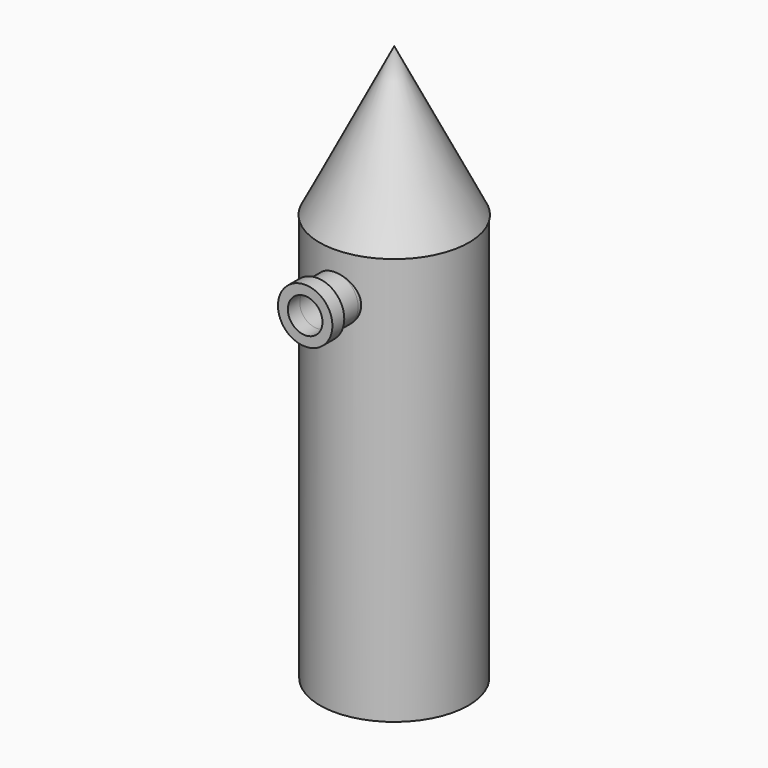
from build123d import *

# Parameters (mm, degrees)
F1_R      = 6.35
F2_DEPTH  = 0.127
F0_R      = 25.4
F3_DEPTH  = 69.85
F6_R      = 6.4657845793
F7_DEPTH  = 152.4
F9_R      = 5.9402933738
F10_DEPTH = 12.7
F9_R_2    = 7.9512438963
F11_DEPTH = 12.7
F12_R     = 9.3192729134
F12_R_2   = 5.9212982026
F13_DEPTH = 5.08
F14_DEPTH = 2.54


with BuildPart() as f2:
    # F1 (on Top) → F2 (new body, symmetric)
    with BuildSketch(Plane.XY):
        Circle(F1_R)
    extrude(amount=F2_DEPTH, both=True)


with BuildPart() as f3:
    # F0 (on Top) → F3 (new body, symmetric)
    with BuildSketch(Plane.XY):
        Circle(F0_R)
    extrude(amount=F3_DEPTH, both=True)

    # F6 (on face) → F7 (cut)
    with BuildSketch(Plane(origin=(0, 0, -69.85), x_dir=(1, 0, 0), z_dir=(0, 0, -1))):
        with Locations((0, 14.7828003392)):
            Circle(F6_R)
    extrude(amount=-F7_DEPTH, mode=Mode.SUBTRACT)

    # F9 (on offset) → F10 (cut)
    with BuildSketch(Plane.XZ.offset(25.4)):
        with Locations((0, 54.8095144331)):
            Circle(F9_R)
    extrude(amount=-F10_DEPTH, mode=Mode.SUBTRACT)


with BuildPart() as f5:
    # F4 (on Right) → F5 (revolve)
    with BuildSketch(Plane.YZ):
        Polygon((-25.6031937897, 88.7221992016), (0, 88.7221992016), (0, 139.5729929209), align=None)
    revolve(axis=Axis((0, 0, 114.1475960612), (0, 0, 1)))


with BuildPart() as f11:
    # F9 (on offset) → F11 (new body)
    with BuildSketch(Plane.XZ.offset(25.4)):
        with Locations((0, 54.8095144331)):
            Circle(F9_R_2)
        with Locations((0, 54.8095144331)):
            Circle(F9_R, mode=Mode.SUBTRACT)
    extrude(amount=F11_DEPTH)

    # F12 (on face) → F13 (join)
    with BuildSketch(Plane.XZ.offset(38.1)):
        with Locations((0, 54.8095144331)):
            Circle(F12_R)
        with Locations((0, 54.8095144331)):
            Circle(F12_R_2, mode=Mode.SUBTRACT)
    extrude(amount=-F13_DEPTH)


with BuildPart() as f14:
    # F14 (new): a face of the model
    f14_faces = [f11.part.faces().sort_by_distance(p)[0] for p in [
        (-7.7263487572, -25.4, 54.8095144331),
    ]]
    extrude(f14_faces, amount=F14_DEPTH)


with BuildPart() as f5_1:
    # F15: moved
    add(f5.part.moved(Location((0, 0, -19.05))))


solid = Compound([f2.part, f3.part, f11.part, f14.part, f5_1.part])
